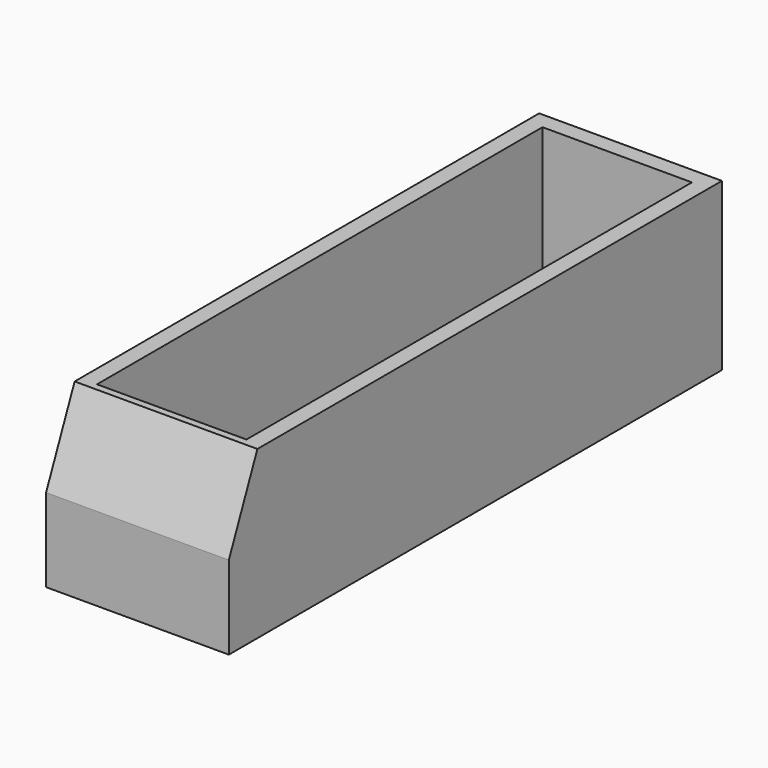
from build123d import *

# Parameters (mm, degrees)
F0_W     = 38.4
F0_H     = 129.5
F0_W_2   = 31.4
F0_H_2   = 111
F1_DEPTH = 2
F2_DEPTH = 35
F3_SIZE2 = 17.5
F3_SIZE  = 7.5
F4_SIZE2 = 32.99999
F4_SIZE  = 5.99999


# Not quite as in the source:
# - a fillet or chamfer is up to 0.001 mm smaller than in the source, because OpenCascade refuses the exact size


with BuildPart() as f1:
    # F0 (on Top) → F1 (new body)
    with BuildSketch(Plane.XY):
        with Locations((0, -5.75)):
            Rectangle(F0_W, F0_H)
        Rectangle(F0_W_2, F0_H_2, mode=Mode.SUBTRACT)
        Rectangle(F0_W_2, F0_H_2)
    extrude(amount=F1_DEPTH)

    # F0 (on Top) → F2 (join)
    with BuildSketch(Plane.XY):
        with Locations((0, -5.75)):
            Rectangle(F0_W, F0_H)
        Rectangle(F0_W_2, F0_H_2, mode=Mode.SUBTRACT)
    extrude(amount=F2_DEPTH)

    # F3
    f3_edges = [f1.edges().sort_by_distance(p)[0] for p in [
        (0, -70.5, 35),
    ]]
    f3_side = f1.faces().sort_by_distance((0, -69.149266, 35))[0]
    chamfer(f3_edges, length=F3_SIZE, length2=F3_SIZE2, reference=f3_side)

    # F4 (size 6 and 33 in the source; OpenCascade refuses exactly that, so slightly less here)
    f4_edges = [f1.edges().sort_by_distance(p)[0] for p in [
        (0, -55.5, 35),
    ]]
    f4_side = f1.faces().sort_by_distance((17.920994, -2, 35))[0]
    chamfer(f4_edges, length=F4_SIZE, length2=F4_SIZE2, reference=f4_side)


solid = f1.part
